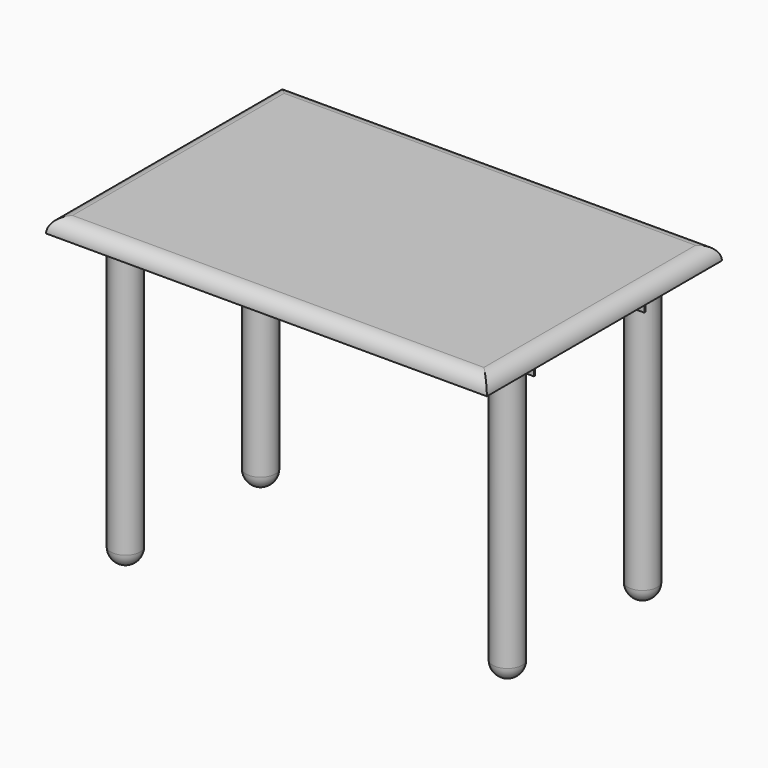
from build123d import *

# Parameters (mm, degrees)
F0_W     = 300
F0_H     = 200
F1_DEPTH = 10
F2_R     = 10
F3_DEPTH = 200
F4_R     = 10
F5_W     = 20
F5_H     = 1
F6_DEPTH = 21
F9_DEPTH = 100
F10_R    = 9.99999


# Not quite as in the source:
# - a fillet or chamfer is up to 0.001 mm smaller than in the source, because OpenCascade refuses the exact size


with BuildPart() as f1:
    # F0 (on Top) → F1 (new body)
    with BuildSketch(Plane.XY):
        with Locations((-5.7550377341, -0.1439023763)):
            Rectangle(F0_W, F0_H)
    extrude(amount=F1_DEPTH)

    # F2 (on face) → F3 (join)
    with BuildSketch(Plane(origin=(0, 0, 0), x_dir=(1, 0, 0), z_dir=(0, 0, -1))):
        with Locations((-125.7550377341, 70.1439023763)):
            Circle(F2_R)
        with Locations((-125.7550377341, -44.8560976237)):
            Circle(F2_R)
        with Locations((114.2449622659, 45.1439023763)):
            Circle(F2_R)
        with Locations((114.2449622659, -69.8560976237)):
            Circle(F2_R)
    extrude(amount=F3_DEPTH)

    # F4
    f4_edges = [f1.edges().sort_by_distance(p)[0] for p in [
        (-135.755038, -70.143902, -200),
        (-135.755038, 44.856098, -200),
        (104.244962, -45.143902, -200),
        (104.244962, 69.856098, -200),
    ]]
    fillet(f4_edges, radius=F4_R)

    # F5 (on face) → F6 (join)
    with BuildSketch(Plane(origin=(0, 0, 0), x_dir=(1, 0, 0), z_dir=(0, 0, -1))):
        with Locations((-125.7550377341, 59.5939023763)):
            Rectangle(F5_W, F5_H)
        with Locations((-125.7550377341, -34.3060976237)):
            Rectangle(F5_W, F5_H)
        with Locations((114.2449622659, -59.3060976237)):
            Rectangle(F5_W, F5_H)
        with Locations((114.2449622659, 34.5939023763)):
            Rectangle(F5_W, F5_H)
    extrude(amount=F6_DEPTH)

    # F7 (on face) + F8 (on face) → F9 (join)
    with BuildSketch(Plane(origin=(0, -59.0939023763, 0), x_dir=(-1, 0, 0), z_dir=(0, 1, 0))):
        with BuildLine():
            ThreePointArc((125.755037734, -21), (132.8261055459, -18.0710678119), (135.7550377341, -11))
            ThreePointArc((135.7550377341, -11), (125.7550377341, -1), (115.7550377341, -11))
            ThreePointArc((115.7550377341, -11), (118.6839699222, -18.0710678119), (125.755037734, -21))
        make_face()
    with BuildSketch(Plane(origin=(0, -34.0939023763, 0), x_dir=(-1, 0, 0), z_dir=(0, 1, 0))):
        with BuildLine():
            ThreePointArc((-114.244962266, -21), (-107.1738944541, -18.0710678119), (-104.2449622659, -11))
            ThreePointArc((-104.2449622659, -11), (-114.2449622659, -1), (-124.2449622659, -11))
            ThreePointArc((-124.2449622659, -11), (-121.3160300778, -18.0710678119), (-114.244962266, -21))
        make_face()
    extrude(amount=F9_DEPTH)

    # F10 (radius 10 in the source; OpenCascade refuses exactly that, so slightly less here)
    f10_edges = [f1.edges().sort_by_distance(p)[0] for p in [
        (-155.755038, -0.143902, 10),
        (-5.755038, 99.856098, 10),
        (144.244962, -0.143902, 10),
        (-5.755038, -100.143902, 10),
    ]]
    fillet(f10_edges, radius=F10_R)


solid = f1.part
